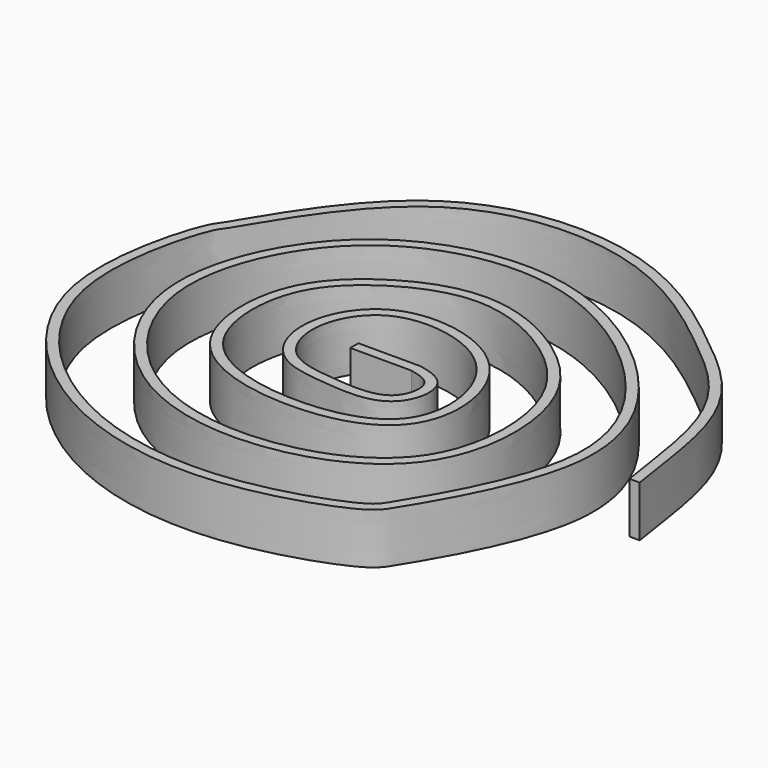
from build123d import *

# Parameters (mm, degrees)
F1_DEPTH = 10


# Not quite as in the source:
# - ends of sketch curves that miss each other by under 0.0002 mm in the source are joined
# - the dataset's text gives a spline's control points without its knots; the knots are read off the source's solid


with BuildPart() as f1:
    # F0 (on Top) → F1 (new body)
    with BuildSketch(Plane.XY):
        with BuildLine():
            Line((-6, 2), (-6, 0))
            Line((-6, 0), (6, 0))
            add(Edge.make_bspline(
                [(6, 0), (7.8240954209, -0.426888851), (11.6213921374, -1.3155614574), (9.9638176776, -10.5190286441), (-2.07008603, -9.5145761805), (-11.9895818193, -8.3298144826), (-16.0389739553, 2.2781838967), (-9.2477320566, 15.0242063021), (9.5001678941, 12.9584512118), (18.492346398, 0.8152895863), (17.5684755683, -15.7617958504), (-2.268301621, -20.6207049063), (-25.5486838625, -14.438413356), (-26.9326847932, 8.2655563439), (-16.7039057291, 19.573220963), (0.1431330638, 27.0324025795), (19.2014115145, 18.0625967688), (30.67531924, 3.0409720829), (28.9726298029, -25.0786767102), (-0.4301579971, -35.4028548605), (-26.9885635344, -27.395766295), (-41.8944184514, -3.0421592088), (-34.3333110863, 21.1340383032), (-18.2451714881, 35.116723691), (7.127142027, 38.4338333637), (33.9019540422, 21.7256396665), (49.4097273291, -5.8042475646), (31.2121054398, -35.5111205129), (28.9224798838, -39.4709828864), (4.1166490444, -48.56138307), (-29.6296982377, -42.3590984627), (-56.2249467546, -12.684513381), (-47.4290580309, 17.6166751374), (-45.1726634984, 19.2721389916), (-28.5254271908, 51.1356440387), (10.6234636787, 53.1306095122), (35.7203479369, 33.6217026833), (51.3819206547, 20.134315786), (53.6970772075, -1.3374801141), (54.6682885973, -7.2114239447)],
                knots=[0, 0, 0, 0, 0.0135818141, 0.0287739971, 0.048897813, 0.0679340831, 0.086731819, 0.1079456658, 0.1325360452, 0.1556379853, 0.1780086006, 0.2039942115, 0.2324620198, 0.2588411109, 0.2822127398, 0.3074405044, 0.3344146165, 0.3606052236, 0.3904385558, 0.422328539, 0.4538532376, 0.4848473857, 0.5143222273, 0.5418343026, 0.5715848946, 0.6052783983, 0.6384954008, 0.6723772539, 0.685621084, 0.7151570799, 0.7512458405, 0.7885428609, 0.8200119597, 0.8308790103, 0.8649723857, 0.9017462881, 0.9354274725, 0.9669697783, 0.9850755448, 0.9850755448, 0.9850755448, 0.9850755448], degree=3))
            Line((54.6682885973, -7.2114239447), (56.6959309989, -7.2114239447))
            add(Edge.make_bspline(
                [(6.4557415069, 1.9473827767), (6.9841434393, 1.8237220892), (7.824526867, 1.6292357232), (8.9873412627, 1.249441733), (9.8713675352, 0.8631705061), (10.7483863049, 0.3217502978), (11.4304082227, -0.3123801391), (11.894623302, -0.9375464318), (12.1900511067, -1.4645195642), (12.4126882526, -2.0138835069), (12.6231092806, -2.757459237), (12.7460781295, -3.7032198746), (12.7085564964, -4.8487108971), (12.5009919207, -5.9926827711), (12.1249556654, -7.1173822278), (11.5720927334, -8.1994798564), (10.9509822461, -9.0381259476), (10.3477373319, -9.6484207001), (9.6747398984, -10.2023778634), (8.7664384767, -10.746561583), (7.6109172065, -11.2056851217), (6.4183936237, -11.5086875302), (5.2001085901, -11.6906756167), (3.551944258, -11.8071814218), (1.8825656644, -11.7779308403), (0.231749072, -11.6700810814), (-0.7812349191, -11.5818393836), (-1.5742536954, -11.5056836021), (-2.3502987964, -11.4286136585), (-3.6954435592, -11.2905762255), (-5.5832974646, -11.0555971435), (-7.7808955053, -10.6194436888), (-9.5455402938, -10.0311531484), (-10.8927866639, -9.3576476549), (-11.8570005678, -8.7366789677), (-12.7598026234, -7.984256419), (-13.5619854533, -7.1287917272), (-14.2666198055, -6.1850810238), (-15.0743953773, -4.8250559205), (-15.83692221, -2.9607852921), (-16.3443386177, -0.5346075259), (-16.4071471149, 1.5910786766), (-16.2242244314, 3.3126709558), (-15.8894632457, 5.02294151), (-15.1912943932, 7.1203795678), (-13.9122228254, 9.4869995688), (-12.1879076432, 11.6096243935), (-10.3813035964, 13.0803412142), (-8.7133472954, 14.0160022582), (-7.3799052757, 14.5715555489), (-5.9920796797, 14.9875079891), (-4.0825265987, 15.3702863822), (-1.6157200957, 15.5481730038), (1.3896103569, 15.33574204), (4.3591161463, 14.7359387933), (7.2099079838, 13.7787913857), (10.7417835487, 12.0447892074), (14.4077681292, 9.0965888643), (17.0135601556, 5.3473087516), (18.4476710161, 2.0133682242), (19.2023538602, -0.6219787106), (19.6285103721, -3.360609568), (19.6864796503, -6.1336279435), (19.3312306028, -8.8760695128), (18.6428129284, -11.0747633839), (17.824063605, -12.7341505699), (17.0697795381, -13.9133599331), (16.1662540857, -15.010611696), (15.142370084, -15.9914134658), (14.0139055153, -16.8636495166), (12.3876034115, -17.8876477624), (10.1546713741, -18.9236792605), (7.2234861165, -19.8226446956), (4.0970775322, -20.4125632811), (0.8287935375, -20.7190293469), (-2.5222653617, -20.7632561561), (-5.9161688294, -20.5575485718), (-9.2951118506, -20.0792580211), (-12.5938922017, -19.3061287136), (-15.7487608864, -18.2109943494), (-18.6927111069, -16.7616925569), (-20.9088525797, -15.2267861971), (-22.4936674491, -13.7840925444), (-23.5762891625, -12.5900292935), (-24.532361312, -11.2868059236), (-25.6216480934, -9.4475964095), (-26.6603253741, -6.9868933959), (-27.4370879404, -3.8808774938), (-27.7893963732, -0.7090750989), (-27.7405361007, 3.496482771), (-26.7814759129, 8.5113293806), (-24.7471537105, 12.6672515124), (-22.5987278315, 15.5206831019), (-20.7649919694, 17.4471482784), (-19.0794062578, 18.89846623), (-17.6505823886, 19.9833327266), (-16.1732153015, 21.0238249122), (-14.2155575045, 22.2563122919), (-11.7077483167, 23.5770783696), (-9.0558451015, 24.6949130708), (-6.2756919942, 25.5612811533), (-3.3848020787, 26.1251206044), (-0.8996117411, 26.299077628), (1.1183669236, 26.2318158893), (3.128333255, 26.03115107), (5.6238636752, 25.5484213142), (8.5610730637, 24.646091515), (11.4157861306, 23.4653174454), (14.1617988432, 22.0476777189), (16.7735770386, 20.4317812165), (19.2210343897, 18.6575392388), (21.4876735921, 16.7521379793), (23.5682889269, 14.6869107404), (25.4416719673, 12.4459424764), (27.0889368342, 10.0134509095), (28.490342002, 7.3773868583), (29.6281138306, 4.5307460196), (30.4887495559, 1.4594145283), (31.0576570426, -1.8148713782), (31.3138773524, -5.2213302994), (31.2330175304, -8.6978392221), (30.7870379745, -12.1785909857), (29.944478287, -15.5968591729), (28.6695654913, -18.8823999271), (27.2165429218, -21.4458429586), (25.7984661268, -23.3482919323), (24.2306724349, -25.1220753351), (22.0168288035, -27.1068877999), (19.0295556225, -29.1272808286), (15.7790254379, -30.8023403122), (11.1763183303, -32.5932917193), (6.289287154, -33.744194355), (1.3447184464, -34.2857288794), (-2.3326829642, -34.391560322), (-5.9517582924, -34.1992562878), (-10.6803212121, -33.5469329566), (-16.3650911808, -31.9929059507), (-21.6314765718, -29.4643523934), (-25.5201575645, -26.8674538232), (-28.2561167744, -24.6335053755), (-30.780997271, -22.1433367564), (-33.836318388, -18.524519718), (-36.3761780624, -14.5184260828), (-38.2972678798, -10.2432579715), (-39.4003500053, -6.9312470315), (-40.0140186405, -4.1082953085), (-40.3048601692, -1.8266936254), (-40.4608130911, 0.4522079429), (-40.4159454111, 3.2884499495), (-39.8774392415, 7.7604482863), (-38.4152740093, 13.1597571359), (-36.1132842492, 18.1409382187), (-33.8888312121, 21.7756901453), (-31.4330883515, 25.1581050623), (-27.9256127874, 28.9066749116), (-23.0416836948, 32.5922561467), (-17.5147542824, 35.4307576409), (-11.389835749, 37.3933244216), (-5.9251134123, 38.2069612436), (-1.417101916, 38.3085019119), (2.010773426, 38.0949993934), (5.4649880156, 37.5780413962), (8.9206955365, 36.7397341449), (12.3382813526, 35.5985278358), (16.8267908034, 33.7043734143), (22.2632884623, 30.6906467681), (27.3509277641, 26.9511203109), (31.1399757575, 23.5995845852), (33.8211306619, 20.9276502379), (36.3302516337, 18.1026580749), (39.3903126734, 14.1206388995), (42.5675470107, 8.7335657845), (44.5593552733, 2.7841598741), (45.2350232496, -2.2934120246), (45.2356586349, -5.5859377551), (44.958508584, -8.2886601793), (44.503792806, -11.0045271548), (43.6477902326, -14.4030708043), (42.2757077818, -18.4177480955), (40.6692406861, -22.2937105025), (38.9357997072, -25.9514626525), (37.1819917793, -29.3082596511), (35.7922626592, -31.7838102477), (34.7773208675, -33.527059477), (34.0781312423, -34.7045178645), (33.5590754722, -35.5670407003), (33.1886886642, -36.1801212893), (32.8530764738, -36.7362857811), (32.4781511496, -37.3567323771), (32.0470918269, -38.0303500328), (31.581381457, -38.6704290699), (31.0377885527, -39.2823962991), (30.4076784729, -39.8430541534), (29.7022833503, -40.3473412014), (28.9071173292, -40.8283905215), (27.9845967113, -41.3232527686), (26.9381013916, -41.8313686867), (25.3817507348, -42.5251208458), (23.1507772142, -43.4125647068), (20.0809861708, -44.4676352335), (16.690571962, -45.4645898212), (13.0532843015, -46.35315782), (9.244019016, -47.0825119139), (4.0317372637, -47.7694767071), (-2.5289110472, -47.9786599973), (-10.3757338719, -47.1690059381), (-16.8055629055, -45.5810515413), (-21.8308655793, -43.7478890604), (-25.5269340879, -42.088088054), (-29.1370075446, -40.1397390392), (-33.8155158964, -37.1544950549), (-39.3080836496, -32.7345878383), (-44.0535863052, -27.4865926125), (-47.2289674337, -22.8425122715), (-49.2545004858, -19.1498655149), (-50.8771971019, -15.260982574), (-51.853335764, -11.8728229937), (-52.3841312723, -9.0779604979), (-52.7396780036, -6.2517530794), (-52.8890766166, -2.709641153), (-52.6930369957, 1.4554810098), (-52.2125776572, 5.4283843808), (-51.5349318368, 9.1027538511), (-50.7450139101, 12.3712210647), (-49.9251184839, 15.1284375252), (-49.2824611398, 16.9171403029), (-48.8206218367, 18.0124981568), (-48.4927620694, 18.6819160359), (-48.1610454152, 19.2484094243), (-47.8416274619, 19.7190096583), (-47.5455684203, 20.1329816212), (-47.2809972624, 20.5146647674), (-47.0339503434, 20.8923007161), (-46.8193030166, 21.2327900528), (-46.5775162122, 21.6254726057), (-46.2214174924, 22.2128053688), (-45.7159506876, 23.0575303678), (-44.7861201782, 24.6130777516), (-43.40591208, 26.8876155646), (-41.42084411, 29.9919040624), (-39.1215728499, 33.3252446556), (-36.5200566875, 36.7441897207), (-33.6254947221, 40.1064502349), (-30.9728163873, 42.7426977612), (-28.707509381, 44.6795632766), (-26.3412139869, 46.4776706901), (-23.2374822822, 48.4033688865), (-19.3357668302, 50.2237818681), (-15.3037331975, 51.5773325004), (-9.8159356284, 52.7941925623), (-4.2489450607, 53.18181905), (1.2307580766, 52.8417538251), (5.2563959867, 52.2466265053), (9.160082715, 51.3346317586), (12.8944649069, 50.1268478246), (16.4449776809, 48.6658344461), (20.9531119969, 46.435360014), (25.140228913, 43.8636118278), (29.0512228301, 41.1105760407), (31.8575371721, 38.9940021715), (34.0991621229, 37.219804965), (35.839736741, 35.8125622323), (37.5454593774, 34.4230491099), (39.6451300963, 32.68565813), (42.8985182937, 29.8082199472), (45.9421652103, 26.6386884525), (48.6382346951, 22.9052741505), (50.1467275471, 20.2883956246), (51.2312511445, 17.9974897329), (51.9800001804, 16.1735475705), (52.6611234549, 14.2385613152), (53.2712832289, 12.1795564499), (53.8080954383, 10.0259869705), (54.444071946, 7.0640037976), (55.1138020013, 3.255199574), (55.790534237, -1.266627968), (56.2972842471, -4.7525345802), (56.5991930185, -6.6369486311), (56.6959309989, -7.2114239447)],
                knots=[0, 0, 0, 0, 0.0039343648, 0.0059015472, 0.0078687296, 0.009835912, 0.0118030944, 0.0127866856, 0.0137702768, 0.014753868, 0.0157374592, 0.0177046416, 0.019671824, 0.0216390064, 0.0236061888, 0.0255733712, 0.0275405536, 0.0285241448, 0.029507736, 0.0314749184, 0.0334421008, 0.0354092832, 0.0373764656, 0.039343648, 0.0432780128, 0.0452451952, 0.0472123776, 0.0481959688, 0.04917956, 0.0511467424, 0.0550811072, 0.059015472, 0.0629498369, 0.0649170193, 0.0668842017, 0.0688513841, 0.0708185665, 0.0727857489, 0.0747529313, 0.0786872961, 0.0826216609, 0.0865560257, 0.0885232081, 0.0904903905, 0.0944247553, 0.0983591201, 0.1022934849, 0.1062278497, 0.1081950321, 0.1101622145, 0.1121293969, 0.1140965793, 0.1180309441, 0.1219653089, 0.1258996737, 0.1298340385, 0.1337684033, 0.1416371329, 0.1495058625, 0.1534402273, 0.1573745921, 0.1613089569, 0.1652433217, 0.1691776865, 0.1731120513, 0.1750792337, 0.1770464161, 0.1790135985, 0.1809807809, 0.1829479634, 0.1849151458, 0.1888495106, 0.1927838754, 0.1967182402, 0.200652605, 0.2045869698, 0.2085213346, 0.2124556994, 0.2163900642, 0.220324429, 0.2242587938, 0.2281931586, 0.230160341, 0.2321275234, 0.2340947058, 0.2360618882, 0.239996253, 0.2439306178, 0.2478649826, 0.2517993474, 0.259668077, 0.2675368066, 0.2714711714, 0.2754055362, 0.279339901, 0.2813070834, 0.2832742658, 0.2872086306, 0.2911429954, 0.2950773602, 0.299011725, 0.3029460898, 0.3068804547, 0.3088476371, 0.3108148195, 0.3147491843, 0.3186835491, 0.3226179139, 0.3265522787, 0.3304866435, 0.3344210083, 0.3383553731, 0.3422897379, 0.3462241027, 0.3501584675, 0.3540928323, 0.3580271971, 0.3619615619, 0.3658959267, 0.3698302915, 0.3737646563, 0.3776990211, 0.3816333859, 0.3855677507, 0.3895021155, 0.3914692979, 0.3934364803, 0.3973708451, 0.4013052099, 0.4052395747, 0.4091739395, 0.4170426691, 0.4209770339, 0.4249113988, 0.4288457636, 0.4327801284, 0.440648858, 0.4485175876, 0.4524519524, 0.4563863172, 0.460320682, 0.4642550468, 0.4721237764, 0.4760581412, 0.479992506, 0.4839268708, 0.4858940532, 0.4878612356, 0.4917956004, 0.4957299652, 0.5035986948, 0.5114674244, 0.5154017892, 0.519336154, 0.5272048836, 0.5350736132, 0.5429423428, 0.5508110725, 0.5586798021, 0.5626141669, 0.5665485317, 0.5704828965, 0.5744172613, 0.5783516261, 0.5822859909, 0.5901547205, 0.5980234501, 0.6019578149, 0.6058921797, 0.6098265445, 0.6137609093, 0.6216296389, 0.6294983685, 0.6334327333, 0.6373670981, 0.6393342805, 0.6413014629, 0.6452358277, 0.6491701925, 0.6531045573, 0.6570389221, 0.6609732869, 0.6649076517, 0.6668748342, 0.6688420166, 0.670809199, 0.6717927902, 0.6727763814, 0.6747435638, 0.6767107462, 0.6786779286, 0.680645111, 0.6826122934, 0.6845794758, 0.6865466582, 0.6885138406, 0.690481023, 0.6924482054, 0.6963825702, 0.700316935, 0.7042512998, 0.7081856646, 0.7121200294, 0.7160543942, 0.7239231238, 0.7317918534, 0.739660583, 0.7435949478, 0.7475293126, 0.7514636774, 0.7553980422, 0.7632667718, 0.7711355014, 0.7750698662, 0.779004231, 0.7829385958, 0.7868729606, 0.7888401431, 0.7908073255, 0.7947416903, 0.7986760551, 0.8026104199, 0.8065447847, 0.8104791495, 0.8144135143, 0.8183478791, 0.8203150615, 0.8222822439, 0.8242494263, 0.8262166087, 0.8281837911, 0.8301509735, 0.8311345647, 0.8321181559, 0.8331017471, 0.8340853383, 0.8360525207, 0.8380197031, 0.8419540679, 0.8458884327, 0.8498227975, 0.8537571623, 0.8576915271, 0.8616258919, 0.8635930743, 0.8655602567, 0.8694946215, 0.8734289863, 0.8773633511, 0.8812977159, 0.8891664455, 0.8931008103, 0.8970351751, 0.9009695399, 0.9049039047, 0.9088382695, 0.9127726344, 0.920641364, 0.9245757288, 0.9285100936, 0.9324444584, 0.9344116408, 0.9363788232, 0.940313188, 0.9442475528, 0.9521162824, 0.9560506472, 0.959985012, 0.9619521944, 0.9639193768, 0.9658865592, 0.9678537416, 0.969820924, 0.9717881064, 0.9757224712, 0.979656836, 0.9835912008, 0.9854189729, 0.9854189729, 0.9854189729, 0.9854189729], degree=3))
            Line((6.4557415069, 1.9473827767), (6, 2))
            Line((6, 2), (-6, 2))
        make_face()
    extrude(amount=F1_DEPTH)


solid = f1.part
